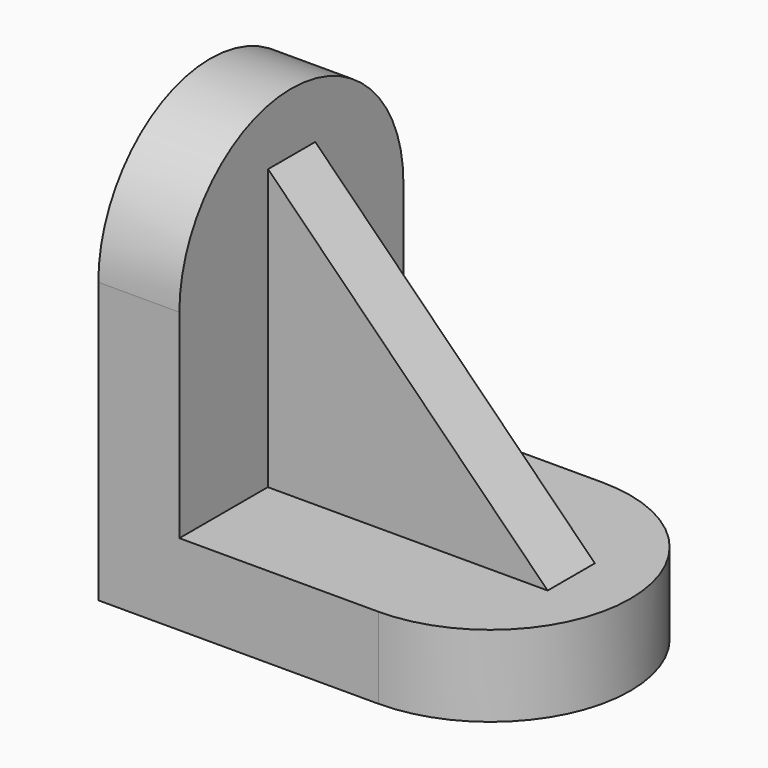
from build123d import *

# Parameters (mm, degrees)
F1_W     = 38
F1_H     = 38
F2_DEPTH = 11
F3_DEPTH = 11
F9_E8_W  = 53.7300702473
F9_E8_H  = 8


with BuildPart() as f2:
    # F1 (on Right) → F2 (new body)
    with BuildSketch(Plane.YZ):
        with Locations((19, 19)):
            Rectangle(F1_W, F1_H)
        with BuildLine():
            ThreePointArc((38, 38), (19, 57), (0, 38))
            Line((0, 38), (38, 38))
        make_face()
    extrude(amount=F2_DEPTH)

    # F0 (on Top) → F3 (join)
    with BuildSketch(Plane.XY):
        with BuildLine():
            Line((0, 38), (0, 0))
            Line((0, 0), (38, 0))
            ThreePointArc((38, 0), (57, 19), (38, 38))
            Line((38, 38), (0, 38))
        make_face()
    extrude(amount=F3_DEPTH)

    # F9_E8 (on explicit) → F10 (join, up to the next surface of F2)
    with BuildSketch(Plane(origin=(11.0387885943, 23, 49), x_dir=(0.7065170626, 0, -0.7076960083), z_dir=(-0.7076960083, 0, -0.7065170626))):
        with Locations((26.8650351237, 4)):
            Rectangle(F9_E8_W, F9_E8_H)
    extrude(until=Until.NEXT)


solid = f2.part
